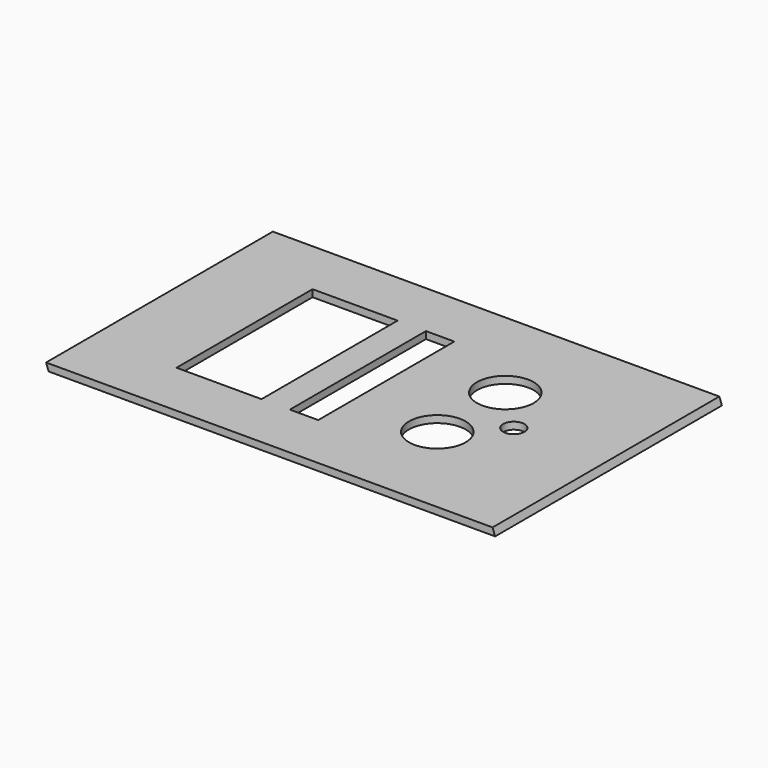
from build123d import *

# Parameters (mm, degrees)
F0_W     = 406.4
F0_H     = 254
F0_R     = 25.4
F0_W_2   = 76.2
F0_H_2   = 152.4
F0_W_3   = 25.4
F0_R_2   = 9.525
F1_DEPTH = 6.35
F3_DEPTH = 254.001
F5_DEPTH = 254.001


with BuildPart() as f1:
    # F0 (on Top) → F1 (new body)
    with BuildSketch(Plane.XY):
        with Locations((203.2, 127)):
            Rectangle(F0_W, F0_H)
        with Locations((279.4, 88.9)):
            Circle(F0_R, mode=Mode.SUBTRACT)
        with Locations((114.3, 127)):
            Rectangle(F0_W_2, F0_H_2, mode=Mode.SUBTRACT)
        with Locations((190.5, 127)):
            Rectangle(F0_W_3, F0_H_2, mode=Mode.SUBTRACT)
        with Locations((279.4, 165.1)):
            Circle(F0_R, mode=Mode.SUBTRACT)
        with Locations((317.5, 127)):
            Circle(F0_R_2, mode=Mode.SUBTRACT)
    extrude(amount=F1_DEPTH)

    # F2 (on face) → F3 (cut, through all)
    with BuildSketch(Plane.XZ):
        Polygon((2.3112109876, 0), (0, 6.35), (0, 0), align=None)
    extrude(amount=-F3_DEPTH, mode=Mode.SUBTRACT)

    # F4 (on face) → F5 (cut, through all)
    with BuildSketch(Plane.XZ):
        Polygon((400.05, 6.35), (402.3612109876, 0), (406.4, 0), (406.4, 6.35), align=None)
        Polygon((396.6623240103, 15.657563286), (400.05, 6.35), (406.4, 6.35), (406.4, 0), (417.733579874, 0), (417.733579874, 15.657563286), align=None)
    extrude(amount=-F5_DEPTH, mode=Mode.SUBTRACT)


solid = f1.part
